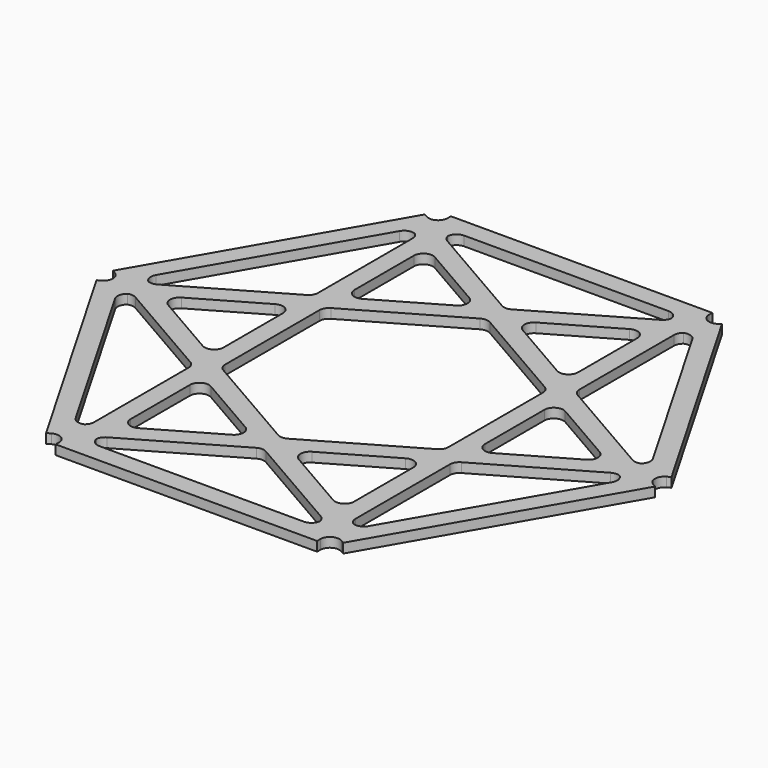
from build123d import *

# Parameters (mm, degrees)
F1_DEPTH    = 2
F2_T1_DEPTH = 2


# Not quite as in the source:
# - a fillet or chamfer that OpenCascade refuses, or shapes differently, is made with other operations: its cross-section is extruded or revolved along the edge and cut away or added


with BuildPart() as f1:
    # F0 (on Top) → F1 (new body)
    with BuildSketch(Plane.XY):
        Polygon((-23.5, 13.567731326), (-27.5, 11.2583302492), (-27.5, -11.2583302492), (-23.5, -13.567731326), align=None)
        Polygon((-23.5, -13.567731326), (-27.5, -11.2583302492), (-27.5, -15.8771324027), (-23.5, -18.1865334795), align=None)
        Polygon((0, -27.1354626519), (-23.5, -13.567731326), (-23.5, -18.1865334795), (-4, -29.4448637287), align=None)
        Polygon((-27.5, -15.8771324027), (-27.5, -11.2583302492), (-47, 0), (-51, -2.3094010768), align=None)
        Polygon((-23.5, -18.1865334795), (-27.5, -15.8771324027), (-27.5, -43.0125950546), (-23.5, -40.7031939779), align=None)
        Polygon((-23.5, -40.7031939779), (-27.5, -43.0125950546), (-27.5, -47.6313972081), (-23.5, -45.3219961314), align=None)
        Polygon((-51, -2.3094010768), (-55, 0), (-58.75, -2.1650635095), (-31.25, -49.7964607176), (-27.5, -47.6313972081), (-27.5, -43.0125950546), (-29.7858983849, -44.3323591025), (-53.2858983849, -3.6291651246), align=None)
        Polygon((-23.5, -45.3219961314), (-27.5, -47.6313972081), (-27.5, -51.9615242271), (27.5, -51.9615242271), (27.5, -47.6313972081), (23.5, -45.3219961314), (23.5, -47.9615242271), (-23.5, -47.9615242271), align=None)
        Polygon((23.5, -40.7031939779), (4, -29.4448637287), (0, -31.7542648054), (23.5, -45.3219961314), align=None)
        Polygon((27.5, -47.6313972081), (27.5, -43.0125950546), (23.5, -40.7031939779), (23.5, -45.3219961314), align=None)
        Polygon((4, -29.4448637287), (0, -27.1354626519), (-4, -29.4448637287), (0, -31.7542648054), align=None)
        Polygon((-4, -29.4448637287), (-23.5, -40.7031939779), (-23.5, -45.3219961314), (0, -31.7542648054), align=None)
        Polygon((23.5, -18.1865334795), (23.5, -13.567731326), (0, -27.1354626519), (4, -29.4448637287), align=None)
        Polygon((27.5, -43.0125950546), (27.5, -15.8771324027), (23.5, -18.1865334795), (23.5, -40.7031939779), align=None)
        Polygon((27.5, -15.8771324027), (27.5, -11.2583302492), (23.5, -13.567731326), (23.5, -18.1865334795), align=None)
        Polygon((58.75, -2.1650635095), (55, 0), (51, -2.3094010768), (53.2858983849, -3.6291651246), (29.7858983849, -44.3323591025), (27.5, -43.0125950546), (27.5, -47.6313972081), (31.25, -49.7964607176), align=None)
        Polygon((47, 0), (27.5, -11.2583302492), (27.5, -15.8771324027), (51, -2.3094010768), align=None)
        Polygon((-47, 0), (-51, 2.3094010768), (-55, 0), (-51, -2.3094010768), align=None)
        Polygon((-27.5, 11.2583302492), (-27.5, 15.8771324027), (-51, 2.3094010768), (-47, 0), align=None)
        Polygon((-27.5, 43.0125950546), (-27.5, 47.6313972081), (-31.25, 49.7964607176), (-58.75, 2.1650635095), (-55, 0), (-51, 2.3094010768), (-53.2858983849, 3.6291651246), (-29.7858983849, 44.3323591025), align=None)
        Polygon((-23.5, 40.7031939779), (-27.5, 43.0125950546), (-27.5, 15.8771324027), (-23.5, 18.1865334795), align=None)
        Polygon((-4, 29.4448637287), (-23.5, 18.1865334795), (-23.5, 13.567731326), (0, 27.1354626519), align=None)
        Polygon((-23.5, 18.1865334795), (-27.5, 15.8771324027), (-27.5, 11.2583302492), (-23.5, 13.567731326), align=None)
        Polygon((0, 31.7542648054), (-23.5, 45.3219961314), (-23.5, 40.7031939779), (-4, 29.4448637287), align=None)
        Polygon((-23.5, 45.3219961314), (-27.5, 47.6313972081), (-27.5, 43.0125950546), (-23.5, 40.7031939779), align=None)
        Polygon((27.5, 51.9615242271), (-27.5, 51.9615242271), (-27.5, 47.6313972081), (-23.5, 45.3219961314), (-23.5, 47.9615242271), (23.5, 47.9615242271), (23.5, 45.3219961314), (27.5, 47.6313972081), align=None)
        Polygon((4, 29.4448637287), (0, 31.7542648054), (-4, 29.4448637287), (0, 27.1354626519), align=None)
        Polygon((23.5, 40.7031939779), (23.5, 45.3219961314), (0, 31.7542648054), (4, 29.4448637287), align=None)
        Polygon((23.5, 18.1865334795), (4, 29.4448637287), (0, 27.1354626519), (23.5, 13.567731326), align=None)
        Polygon((27.5, 15.8771324027), (27.5, 43.0125950546), (23.5, 40.7031939779), (23.5, 18.1865334795), align=None)
        Polygon((27.5, 43.0125950546), (27.5, 47.6313972081), (23.5, 45.3219961314), (23.5, 40.7031939779), align=None)
        Polygon((31.25, 49.7964607176), (27.5, 47.6313972081), (27.5, 43.0125950546), (29.7858983849, 44.3323591025), (53.2858983849, 3.6291651246), (51, 2.3094010768), (55, 0), (58.75, 2.1650635095), align=None)
        Polygon((27.5, 11.2583302492), (27.5, 15.8771324027), (23.5, 18.1865334795), (23.5, 13.567731326), align=None)
        Polygon((27.5, -11.2583302492), (27.5, 11.2583302492), (23.5, 13.567731326), (23.5, -13.567731326), align=None)
        Polygon((51, 2.3094010768), (27.5, 15.8771324027), (27.5, 11.2583302492), (47, 0), align=None)
        Polygon((55, 0), (51, 2.3094010768), (47, 0), (51, -2.3094010768), align=None)
    extrude(amount=F1_DEPTH)

    # F2: fillet of radius 2 on 60 edges, made by hand

    # F2_s2 → F2_t1 (join)
    with BuildSketch(Plane.XY):
        with BuildLine():
            ThreePointArc((-23.5, 45.9615242271), (-22.9142135624, 47.3757377894), (-21.5, 47.9615242271))
            Line((-21.5, 47.9615242271), (-23.5, 47.9615242271))
            Line((-23.5, 47.9615242271), (-23.5, 45.9615242271))
        make_face()
        with BuildLine():
            ThreePointArc((-30.7858983849, 42.6003082949), (-29.5714856675, 43.5321599475), (-28.0538475773, 43.3323591025))
            Line((-28.0538475773, 43.3323591025), (-29.7858983849, 44.3323591025))
            Line((-29.7858983849, 44.3323591025), (-30.7858983849, 42.6003082949))
        make_face()
        with BuildLine():
            ThreePointArc((-23.5, 37.2390923627), (-22.5, 38.9711431703), (-20.5, 38.9711431703))
            Line((-20.5, 38.9711431703), (-23.5, 40.7031939779))
            Line((-23.5, 40.7031939779), (-23.5, 37.2390923627))
        make_face()
        with BuildLine():
            ThreePointArc((-23.5, 12.4130307876), (-23.2320508076, 13.4130307876), (-22.5, 14.1450815951))
            Line((-22.5, 14.1450815951), (-23.5, 13.567731326))
            Line((-23.5, 13.567731326), (-23.5, 12.4130307876))
        make_face()
        with BuildLine():
            ThreePointArc((-1, 26.5581123827), (0, 26.8260615752), (1, 26.5581123827))
            Line((1, 26.5581123827), (0, 27.1354626519))
            Line((0, 27.1354626519), (-1, 26.5581123827))
        make_face()
        with BuildLine():
            ThreePointArc((21.5, 47.9615242271), (22.9142135624, 47.3757377894), (23.5, 45.9615242271))
            Line((23.5, 45.9615242271), (23.5, 47.9615242271))
            Line((23.5, 47.9615242271), (21.5, 47.9615242271))
        make_face()
        with BuildLine():
            ThreePointArc((20.5, 38.9711431703), (22.5, 38.9711431703), (23.5, 37.2390923627))
            Line((23.5, 37.2390923627), (23.5, 40.7031939779))
            Line((23.5, 40.7031939779), (20.5, 38.9711431703))
        make_face()
        with BuildLine():
            ThreePointArc((28.0538475773, 43.3323591025), (29.5714856675, 43.5321599475), (30.7858983849, 42.6003082949))
            Line((30.7858983849, 42.6003082949), (29.7858983849, 44.3323591025))
            Line((29.7858983849, 44.3323591025), (28.0538475773, 43.3323591025))
        make_face()
        with BuildLine():
            ThreePointArc((22.5, 14.1450815951), (23.2320508076, 13.4130307876), (23.5, 12.4130307876))
            Line((23.5, 12.4130307876), (23.5, 13.567731326))
            Line((23.5, 13.567731326), (22.5, 14.1450815951))
        make_face()
        with BuildLine():
            ThreePointArc((-27.5, 7.7942286341), (-28.5, 9.5262794416), (-30.5, 9.5262794416))
            Line((-30.5, 9.5262794416), (-27.5, 11.2583302492))
            Line((-27.5, 11.2583302492), (-27.5, 7.7942286341))
        make_face()
        with BuildLine():
            ThreePointArc((-27.5, -17.0318329411), (-27.7679491924, -16.0318329411), (-28.5, -15.2997821335))
            Line((-28.5, -15.2997821335), (-27.5, -15.8771324027))
            Line((-27.5, -15.8771324027), (-27.5, -17.0318329411))
        make_face()
        with BuildLine():
            ThreePointArc((-52.2858983849, -5.3612159322), (-52.4856992299, -3.843577842), (-51.5538475773, -2.6291651246))
            Line((-51.5538475773, -2.6291651246), (-53.2858983849, -3.6291651246))
            Line((-53.2858983849, -3.6291651246), (-52.2858983849, -5.3612159322))
        make_face()
        with BuildLine():
            ThreePointArc((-44, -1.7320508076), (-45, 0), (-44, 1.7320508076))
            Line((-44, 1.7320508076), (-47, 0))
            Line((-47, 0), (-44, -1.7320508076))
        make_face()
        with BuildLine():
            ThreePointArc((-51.5538475773, 2.6291651246), (-52.4856992299, 3.843577842), (-52.2858983849, 5.3612159322))
            Line((-52.2858983849, 5.3612159322), (-53.2858983849, 3.6291651246))
            Line((-53.2858983849, 3.6291651246), (-51.5538475773, 2.6291651246))
        make_face()
        with BuildLine():
            ThreePointArc((-23.5, -12.4130307876), (-23.2320508076, -13.4130307876), (-22.5, -14.1450815951))
            Line((-22.5, -14.1450815951), (-23.5, -13.567731326))
            Line((-23.5, -13.567731326), (-23.5, -12.4130307876))
        make_face()
        with BuildLine():
            ThreePointArc((-28.0538475773, -43.3323591025), (-29.5714856675, -43.5321599475), (-30.7858983849, -42.6003082949))
            Line((-30.7858983849, -42.6003082949), (-29.7858983849, -44.3323591025))
            Line((-29.7858983849, -44.3323591025), (-28.0538475773, -43.3323591025))
        make_face()
        with BuildLine():
            ThreePointArc((-20.5, -38.9711431703), (-22.5, -38.9711431703), (-23.5, -37.2390923627))
            Line((-23.5, -37.2390923627), (-23.5, -40.7031939779))
            Line((-23.5, -40.7031939779), (-20.5, -38.9711431703))
        make_face()
        with BuildLine():
            ThreePointArc((-21.5, -47.9615242271), (-22.9142135624, -47.3757377894), (-23.5, -45.9615242271))
            Line((-23.5, -45.9615242271), (-23.5, -47.9615242271))
            Line((-23.5, -47.9615242271), (-21.5, -47.9615242271))
        make_face()
        with BuildLine():
            ThreePointArc((1, -26.5581123827), (0, -26.8260615752), (-1, -26.5581123827))
            Line((-1, -26.5581123827), (0, -27.1354626519))
            Line((0, -27.1354626519), (1, -26.5581123827))
        make_face()
        with BuildLine():
            ThreePointArc((27.5, 7.7942286341), (28.5, 9.5262794416), (30.5, 9.5262794416))
            Line((30.5, 9.5262794416), (27.5, 11.2583302492))
            Line((27.5, 11.2583302492), (27.5, 7.7942286341))
        make_face()
        with BuildLine():
            ThreePointArc((27.5, -17.0318329411), (27.7679491924, -16.0318329411), (28.5, -15.2997821335))
            Line((28.5, -15.2997821335), (27.5, -15.8771324027))
            Line((27.5, -15.8771324027), (27.5, -17.0318329411))
        make_face()
        with BuildLine():
            ThreePointArc((50, -2.8867513459), (51, -2.6188021535), (52, -2.8867513459))
            Line((52, -2.8867513459), (51, -2.3094010768))
            Line((51, -2.3094010768), (50, -2.8867513459))
        make_face()
        with BuildLine():
            ThreePointArc((51.5538475773, -2.6291651246), (52.4856992299, -3.843577842), (52.2858983849, -5.3612159322))
            Line((52.2858983849, -5.3612159322), (53.2858983849, -3.6291651246))
            Line((53.2858983849, -3.6291651246), (51.5538475773, -2.6291651246))
        make_face()
        with BuildLine():
            ThreePointArc((52.2858983849, 5.3612159322), (52.4856992299, 3.843577842), (51.5538475773, 2.6291651246))
            Line((51.5538475773, 2.6291651246), (53.2858983849, 3.6291651246))
            Line((53.2858983849, 3.6291651246), (52.2858983849, 5.3612159322))
        make_face()
        with BuildLine():
            ThreePointArc((44, 1.7320508076), (45, 0), (44, -1.7320508076))
            Line((44, -1.7320508076), (47, 0))
            Line((47, 0), (44, 1.7320508076))
        make_face()
        with BuildLine():
            ThreePointArc((27.5, 41.8578945162), (27.7679491924, 42.8578945162), (28.5, 43.5899453238))
            Line((28.5, 43.5899453238), (27.5, 43.0125950546))
            Line((27.5, 43.0125950546), (27.5, 41.8578945162))
        make_face()
        with BuildLine():
            ThreePointArc((22.5, 44.7446458622), (23.2320508076, 45.4766966698), (23.5, 46.4766966698))
            Line((23.5, 46.4766966698), (23.5, 45.3219961314))
            Line((23.5, 45.3219961314), (22.5, 44.7446458622))
        make_face()
        with BuildLine():
            ThreePointArc((-22.5, 44.7446458622), (-23.2320508076, 45.4766966698), (-23.5, 46.4766966698))
            Line((-23.5, 46.4766966698), (-23.5, 45.3219961314))
            Line((-23.5, 45.3219961314), (-22.5, 44.7446458622))
        make_face()
        with BuildLine():
            ThreePointArc((-50, 2.8867513459), (-51, 2.6188021535), (-52, 2.8867513459))
            Line((-52, 2.8867513459), (-51, 2.3094010768))
            Line((-51, 2.3094010768), (-50, 2.8867513459))
        make_face()
        with BuildLine():
            ThreePointArc((-20.5, 19.918584287), (-22.5, 19.918584287), (-23.5, 21.6506350946))
            Line((-23.5, 21.6506350946), (-23.5, 18.1865334795))
            Line((-23.5, 18.1865334795), (-20.5, 19.918584287))
        make_face()
        with BuildLine():
            ThreePointArc((1, 32.3316150746), (0, 32.0636658822), (-1, 32.3316150746))
            Line((-1, 32.3316150746), (0, 31.7542648054))
            Line((0, 31.7542648054), (1, 32.3316150746))
        make_face()
        with BuildLine():
            ThreePointArc((-27.5, 17.0318329411), (-27.7679491924, 16.0318329411), (-28.5, 15.2997821335))
            Line((-28.5, 15.2997821335), (-27.5, 15.8771324027))
            Line((-27.5, 15.8771324027), (-27.5, 17.0318329411))
        make_face()
        with BuildLine():
            ThreePointArc((-7, 27.7128129211), (-6, 29.4448637287), (-7, 31.1769145362))
            Line((-7, 31.1769145362), (-4, 29.4448637287))
            Line((-4, 29.4448637287), (-7, 27.7128129211))
        make_face()
        with BuildLine():
            ThreePointArc((23.5, -12.4130307876), (23.2320508076, -13.4130307876), (22.5, -14.1450815951))
            Line((22.5, -14.1450815951), (23.5, -13.567731326))
            Line((23.5, -13.567731326), (23.5, -12.4130307876))
        make_face()
        with BuildLine():
            ThreePointArc((20.5, 19.918584287), (22.5, 19.918584287), (23.5, 21.6506350946))
            Line((23.5, 21.6506350946), (23.5, 18.1865334795))
            Line((23.5, 18.1865334795), (20.5, 19.918584287))
        make_face()
        with BuildLine():
            ThreePointArc((20.5, -38.9711431703), (22.5, -38.9711431703), (23.5, -37.2390923627))
            Line((23.5, -37.2390923627), (23.5, -40.7031939779))
            Line((23.5, -40.7031939779), (20.5, -38.9711431703))
        make_face()
        with BuildLine():
            ThreePointArc((23.5, -45.9615242271), (22.9142135624, -47.3757377894), (21.5, -47.9615242271))
            Line((21.5, -47.9615242271), (23.5, -47.9615242271))
            Line((23.5, -47.9615242271), (23.5, -45.9615242271))
        make_face()
        with BuildLine():
            ThreePointArc((30.7858983849, -42.6003082949), (29.5714856675, -43.5321599475), (28.0538475773, -43.3323591025))
            Line((28.0538475773, -43.3323591025), (29.7858983849, -44.3323591025))
            Line((29.7858983849, -44.3323591025), (30.7858983849, -42.6003082949))
        make_face()
        with BuildLine():
            ThreePointArc((-20.5, -19.918584287), (-22.5, -19.918584287), (-23.5, -21.6506350946))
            Line((-23.5, -21.6506350946), (-23.5, -18.1865334795))
            Line((-23.5, -18.1865334795), (-20.5, -19.918584287))
        make_face()
        with BuildLine():
            ThreePointArc((-1, -32.3316150746), (0, -32.0636658822), (1, -32.3316150746))
            Line((1, -32.3316150746), (0, -31.7542648054))
            Line((0, -31.7542648054), (-1, -32.3316150746))
        make_face()
        with BuildLine():
            ThreePointArc((-7, -27.7128129211), (-6, -29.4448637287), (-7, -31.1769145362))
            Line((-7, -31.1769145362), (-4, -29.4448637287))
            Line((-4, -29.4448637287), (-7, -27.7128129211))
        make_face()
        with BuildLine():
            ThreePointArc((-27.5, -41.8578945162), (-27.7679491924, -42.8578945162), (-28.5, -43.5899453238))
            Line((-28.5, -43.5899453238), (-27.5, -43.0125950546))
            Line((-27.5, -43.0125950546), (-27.5, -41.8578945162))
        make_face()
        with BuildLine():
            ThreePointArc((-27.5, -7.7942286341), (-28.5, -9.5262794416), (-30.5, -9.5262794416))
            Line((-30.5, -9.5262794416), (-27.5, -11.2583302492))
            Line((-27.5, -11.2583302492), (-27.5, -7.7942286341))
        make_face()
        with BuildLine():
            ThreePointArc((-27.5, 41.8578945162), (-27.7679491924, 42.8578945162), (-28.5, 43.5899453238))
            Line((-28.5, 43.5899453238), (-27.5, 43.0125950546))
            Line((-27.5, 43.0125950546), (-27.5, 41.8578945162))
        make_face()
        with BuildLine():
            ThreePointArc((27.5, 17.0318329411), (27.7679491924, 16.0318329411), (28.5, 15.2997821335))
            Line((28.5, 15.2997821335), (27.5, 15.8771324027))
            Line((27.5, 15.8771324027), (27.5, 17.0318329411))
        make_face()
        with BuildLine():
            ThreePointArc((52, 2.8867513459), (51, 2.6188021535), (50, 2.8867513459))
            Line((50, 2.8867513459), (51, 2.3094010768))
            Line((51, 2.3094010768), (52, 2.8867513459))
        make_face()
        with BuildLine():
            ThreePointArc((27.5, -41.8578945162), (27.7679491924, -42.8578945162), (28.5, -43.5899453238))
            Line((28.5, -43.5899453238), (27.5, -43.0125950546))
            Line((27.5, -43.0125950546), (27.5, -41.8578945162))
        make_face()
        with BuildLine():
            ThreePointArc((22.5, -44.7446458622), (23.2320508076, -45.4766966698), (23.5, -46.4766966698))
            Line((23.5, -46.4766966698), (23.5, -45.3219961314))
            Line((23.5, -45.3219961314), (22.5, -44.7446458622))
        make_face()
        with BuildLine():
            ThreePointArc((-22.5, -44.7446458622), (-23.2320508076, -45.4766966698), (-23.5, -46.4766966698))
            Line((-23.5, -46.4766966698), (-23.5, -45.3219961314))
            Line((-23.5, -45.3219961314), (-22.5, -44.7446458622))
        make_face()
        with BuildLine():
            ThreePointArc((-30.5, -49.3634480157), (-28.5, -49.3634480157), (-27.5, -51.0954988233))
            Line((-27.5, -51.0954988233), (-27.5, -47.6313972081))
            Line((-27.5, -47.6313972081), (-30.5, -49.3634480157))
        make_face()
        with BuildLine():
            ThreePointArc((27.5, -51.0954988233), (28.5, -49.3634480157), (30.5, -49.3634480157))
            Line((30.5, -49.3634480157), (27.5, -47.6313972081))
            Line((27.5, -47.6313972081), (27.5, -51.0954988233))
        make_face()
        with BuildLine():
            ThreePointArc((58, -1.7320508076), (57, 0), (58, 1.7320508076))
            Line((58, 1.7320508076), (55, 0))
            Line((55, 0), (58, -1.7320508076))
        make_face()
        with BuildLine():
            ThreePointArc((30.5, 49.3634480157), (28.5, 49.3634480157), (27.5, 51.0954988233))
            Line((27.5, 51.0954988233), (27.5, 47.6313972081))
            Line((27.5, 47.6313972081), (30.5, 49.3634480157))
        make_face()
        with BuildLine():
            ThreePointArc((-30.5, 49.3634480157), (-28.5, 49.3634480157), (-27.5, 51.0954988233))
            Line((-27.5, 51.0954988233), (-27.5, 47.6313972081))
            Line((-27.5, 47.6313972081), (-30.5, 49.3634480157))
        make_face()
        with BuildLine():
            ThreePointArc((-58, 1.7320508076), (-57, 0), (-58, -1.7320508076))
            Line((-58, -1.7320508076), (-55, 0))
            Line((-55, 0), (-58, 1.7320508076))
        make_face()
        with BuildLine():
            ThreePointArc((20.5, -19.918584287), (22.5, -19.918584287), (23.5, -21.6506350946))
            Line((23.5, -21.6506350946), (23.5, -18.1865334795))
            Line((23.5, -18.1865334795), (20.5, -19.918584287))
        make_face()
        with BuildLine():
            ThreePointArc((7, -31.1769145362), (6, -29.4448637287), (7, -27.7128129211))
            Line((7, -27.7128129211), (4, -29.4448637287))
            Line((4, -29.4448637287), (7, -31.1769145362))
        make_face()
        with BuildLine():
            ThreePointArc((27.5, -7.7942286341), (28.5, -9.5262794416), (30.5, -9.5262794416))
            Line((30.5, -9.5262794416), (27.5, -11.2583302492))
            Line((27.5, -11.2583302492), (27.5, -7.7942286341))
        make_face()
        with BuildLine():
            ThreePointArc((7, 27.7128129211), (6, 29.4448637287), (7, 31.1769145362))
            Line((7, 31.1769145362), (4, 29.4448637287))
            Line((4, 29.4448637287), (7, 27.7128129211))
        make_face()
        with BuildLine():
            ThreePointArc((-52, -2.8867513459), (-51, -2.6188021535), (-50, -2.8867513459))
            Line((-50, -2.8867513459), (-51, -2.3094010768))
            Line((-51, -2.3094010768), (-52, -2.8867513459))
        make_face()
    extrude(amount=F2_T1_DEPTH)


solid = f1.part
